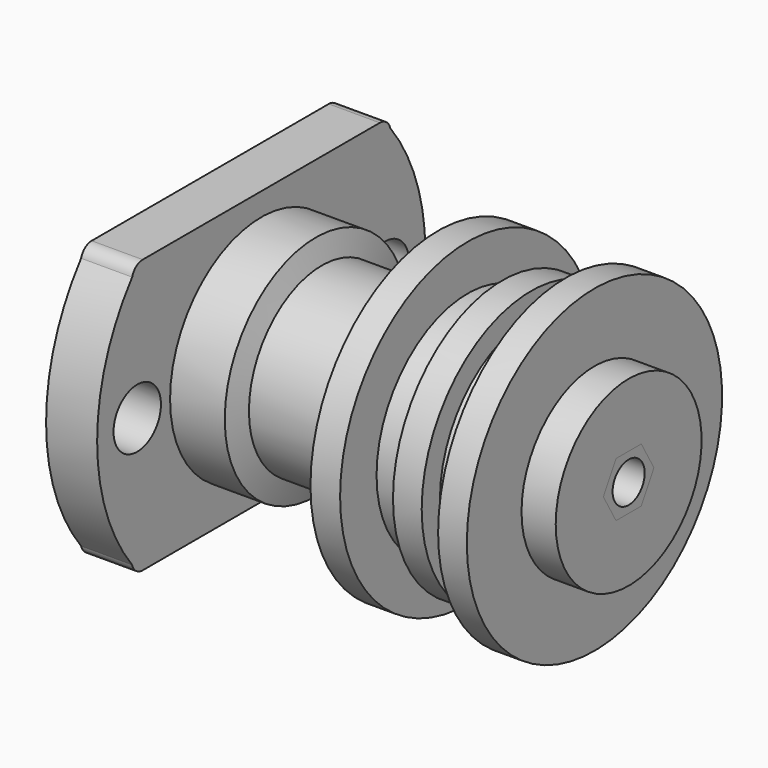
from build123d import *

# Parameters (mm, degrees)
F2_R     = 6.5
F2_R_2   = 25
F3_DEPTH = 11.2
F5_DEPTH = 25
F7_D     = 8.8
F7_DEPTH = 10
F7_TIP   = 2.6437867237


with BuildPart() as f1:
    # F0 (on Top) → F1 (revolve)
    with BuildSketch(Plane.XY):
        Polygon((11.2, 0), (11.2, -25), (23.2, -25), (24.5, -20), (50, -20), (50, -35), (56.5, -35), (56.5, -25), (64.1, -25), (64.1, -30), (70.4, -30), (70.4, -25), (78, -25), (78, -35), (84.3, -35), (84.3, -20), (91.8, -20), (91.8, 0), align=None)
    revolve(axis=Axis((46.0906531856, 0, 0), (-1, 0, 0)))

    # F2 (on face) → F3 (join)
    with BuildSketch(Plane(origin=(11.2, 0, 0), x_dir=(0, -1, 0), z_dir=(-1, 0, 0))):
        with BuildLine():
            Line((32.5, 30), (0, 30))
            Line((0, 30), (-32.5, 30))
            ThreePointArc((-32.5, 30), (-34.3210259826, 29.3840856467), (-35.3943212715, 27.7892429139))
            ThreePointArc((-35.3943212715, 27.7892429139), (-45, 0), (-35.3943212715, -27.7892429139))
            ThreePointArc((-35.3943212715, -27.7892429139), (-34.3210259826, -29.3840856467), (-32.5, -30))
            Line((-32.5, -30), (0, -30))
            Line((0, -30), (32.5, -30))
            ThreePointArc((32.5, -30), (34.3210259826, -29.3840856467), (35.3943212715, -27.7892429139))
            ThreePointArc((35.3943212715, -27.7892429139), (45, 0), (35.3943212715, 27.7892429139))
            ThreePointArc((35.3943212715, 27.7892429139), (34.3210259826, 29.3840856467), (32.5, 30))
        make_face()
        with Locations((-34, 0)):
            Circle(F2_R, mode=Mode.SUBTRACT)
        Circle(F2_R_2, mode=Mode.SUBTRACT)
        with Locations((34, 0)):
            Circle(F2_R, mode=Mode.SUBTRACT)
        Circle(F2_R_2)
    extrude(amount=F3_DEPTH)


with BuildPart() as f5:
    # F4 (on face) → F5 (new body)
    with BuildSketch(Plane.YZ.offset(91.8)):
        Polygon((-3.4641016151, -6), (3.4641016151, -6), (6.9282032303, 0), (3.4641016151, 6), (-3.4641016151, 6), (-6.9282032303, 0), align=None)
    extrude(amount=-F5_DEPTH)


with BuildPart() as f1_1:
    add(f1.part)

    # F6: cut F5
    add(f5.part, mode=Mode.SUBTRACT)


with BuildPart() as f5_1:
    add(f5.part)

    # F7
    with Locations(Plane.YZ.offset(91.8)):
        with Locations((0, 0)):
            Hole(F7_D / 2, depth=F7_DEPTH)
            with Locations((0, 0, -(F7_DEPTH + F7_TIP / 2))):  # 118° drill point
                Cone(0, F7_D / 2, F7_TIP, mode=Mode.SUBTRACT)


solid = Compound([f1_1.part, f5_1.part])
